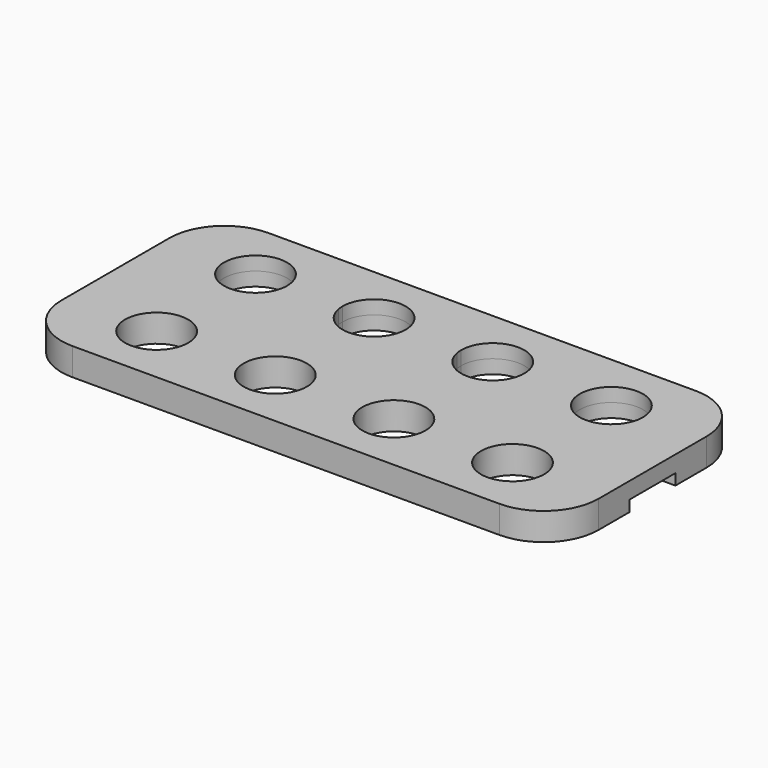
from build123d import *

# Parameters (mm, degrees)
F1_DEPTH = 2.5
F2_DEPTH = 2.5
F3_DEPTH = 0.5
F4_R     = 10


# Not quite as in the source:
# - a feature names something its author has since deleted; it is built from what else it names


with BuildPart() as f1:
    # F0 (on Top) → F1 (new body, symmetric)
    with BuildSketch(Plane.XY):
        with BuildLine():
            Line((-41.7, 5.2), (-3.6, 5.2))
            Line((-3.6, 5.2), (-3.6, 5.5))
            ThreePointArc((-3.6, 5.5), (-7.2954363748, 6.8447474533), (-9.2623758265, 10.25))
            Line((-9.2623758265, 10.25), (-19.5376241735, 10.25))
            ThreePointArc((-19.5376241735, 10.25), (-30.9280520686, 11.7519158285), (-19.45, 11.25))
            Line((-19.45, 11.25), (-9.35, 11.25))
            ThreePointArc((-9.35, 11.25), (-3.6, 17), (2.15, 11.25))
            Line((2.15, 11.25), (7.2, 11.25))
            Line((7.2, 11.25), (12.25, 11.25))
            ThreePointArc((12.25, 11.25), (18, 17), (23.75, 11.25))
            ThreePointArc((23.75, 11.25), (18.5019158285, 5.5219479314), (12.3376241735, 10.25))
            Line((12.3376241735, 10.25), (7.2, 10.25))
            Line((7.2, 10.25), (7.2, 5.2))
            Line((7.2, 5.2), (56.1, 5.2))
            Line((56.1, 5.2), (56.1, 22.3))
            Line((56.1, 22.3), (-41.7, 22.3))
            Line((-41.7, 22.3), (-41.7, 5.2))
        make_face()
        with BuildLine():
            ThreePointArc((45.35, 11.25), (39.6, 5.5), (33.85, 11.25))
            ThreePointArc((33.85, 11.25), (39.6, 17), (45.35, 11.25))
        make_face(mode=Mode.SUBTRACT)
        with BuildLine():
            Line((-3.6, 5.5), (-3.6, 5.2))
            Line((-3.6, 5.2), (7.2, 5.2))
            Line((7.2, 5.2), (7.2, 10.25))
            Line((7.2, 10.25), (2.0623758265, 10.25))
            ThreePointArc((2.0623758265, 10.25), (0.0954363748, 6.8447474533), (-3.6, 5.5))
        make_face()
        with BuildLine():
            Line((-19.5376241735, 10.25), (-9.2623758265, 10.25))
            ThreePointArc((-9.2623758265, 10.25), (-9.3280520686, 10.7480841715), (-9.35, 11.25))
            Line((-9.35, 11.25), (-19.45, 11.25))
            ThreePointArc((-19.45, 11.25), (-19.4719479314, 10.7480841715), (-19.5376241735, 10.25))
        make_face()
        with BuildLine():
            ThreePointArc((2.15, 11.25), (2.1280520686, 10.7480841715), (2.0623758265, 10.25))
            Line((2.0623758265, 10.25), (7.2, 10.25))
            Line((7.2, 10.25), (7.2, 11.25))
            Line((7.2, 11.25), (2.15, 11.25))
        make_face()
        with BuildLine():
            Line((7.2, 11.25), (7.2, 10.25))
            Line((7.2, 10.25), (12.3376241735, 10.25))
            ThreePointArc((12.3376241735, 10.25), (12.2719479314, 10.7480841715), (12.25, 11.25))
            Line((12.25, 11.25), (7.2, 11.25))
        make_face()
    extrude(amount=F1_DEPTH, both=True)



with BuildPart() as f1b:
    # F0 (on Top) → F1, piece 2 (new body, symmetric)
    with BuildSketch(Plane.XY):
        Polygon((56.1, -5.2), (-3.6, -5.2), (-41.7, -5.2), (-41.7, -22.3), (56.1, -22.3), align=None)
        with BuildLine():
            ThreePointArc((-9.2623758265, -10.25), (-7.2954363748, -6.8447474533), (-3.6, -5.5))
            ThreePointArc((-3.6, -5.5), (0.0954363748, -6.8447474533), (2.0623758265, -10.25))
            Line((2.0623758265, -10.25), (12.3376241735, -10.25))
            ThreePointArc((12.3376241735, -10.25), (18.5019158285, -5.5219479314), (23.75, -11.25))
            ThreePointArc((23.75, -11.25), (18, -17), (12.25, -11.25))
            Line((12.25, -11.25), (2.15, -11.25))
            ThreePointArc((2.15, -11.25), (-3.6, -17), (-9.35, -11.25))
            Line((-9.35, -11.25), (-19.45, -11.25))
            ThreePointArc((-19.45, -11.25), (-30.9280520686, -11.7519158285), (-19.5376241735, -10.25))
            Line((-19.5376241735, -10.25), (-9.2623758265, -10.25))
        make_face(mode=Mode.SUBTRACT)
        with BuildLine():
            ThreePointArc((45.35, -11.25), (39.6, -17), (33.85, -11.25))
            ThreePointArc((33.85, -11.25), (39.6, -5.5), (45.35, -11.25))
        make_face(mode=Mode.SUBTRACT)
        with BuildLine():
            Line((12.3376241735, -10.25), (2.0623758265, -10.25))
            ThreePointArc((2.0623758265, -10.25), (2.1280520686, -10.7480841715), (2.15, -11.25))
            Line((2.15, -11.25), (12.25, -11.25))
            ThreePointArc((12.25, -11.25), (12.2719479314, -10.7480841715), (12.3376241735, -10.25))
        make_face()
        with BuildLine():
            ThreePointArc((-9.35, -11.25), (-9.3280520686, -10.7480841715), (-9.2623758265, -10.25))
            Line((-9.2623758265, -10.25), (-19.5376241735, -10.25))
            ThreePointArc((-19.5376241735, -10.25), (-19.4719479314, -10.7480841715), (-19.45, -11.25))
            Line((-19.45, -11.25), (-9.35, -11.25))
        make_face()
    extrude(amount=F1_DEPTH, both=True)


with BuildPart() as f1_1:
    add(f1.part)

    add(f1b.part)  # F2 merges F1b
    # F0 (on Top) → F2 (join)
    with BuildSketch(Plane.XY):
        Polygon((-3.6, -5.2), (-3.6, 0), (-3.6, 5.2), (-41.7, 5.2), (-41.7, -5.2), align=None)
        Polygon((-3.6, 5.2), (-3.6, 0), (-3.6, -5.2), (56.1, -5.2), (56.1, 0), (56.1, 5.2), (7.2, 5.2), align=None)
    extrude(amount=F2_DEPTH)

    # F0 (on Top) → F3 (join)
    with BuildSketch(Plane.XY):
        Polygon((-3.6, 5.2), (-3.6, 0), (-3.6, -5.2), (56.1, -5.2), (56.1, 0), (56.1, 5.2), (7.2, 5.2), align=None)
        Polygon((-3.6, -5.2), (-3.6, 0), (-3.6, 5.2), (-41.7, 5.2), (-41.7, -5.2), align=None)
    extrude(amount=-F3_DEPTH)

    # F4
    f4_edges = [f1_1.edges().sort_by_distance(p)[0] for p in [
        (56.1, -22.3, 0),
        (-41.7, -22.3, 0),
        (-41.7, 22.3, 0),
        (56.1, 22.3, 0),
    ]]
    fillet(f4_edges, radius=F4_R)


solid = f1_1.part
